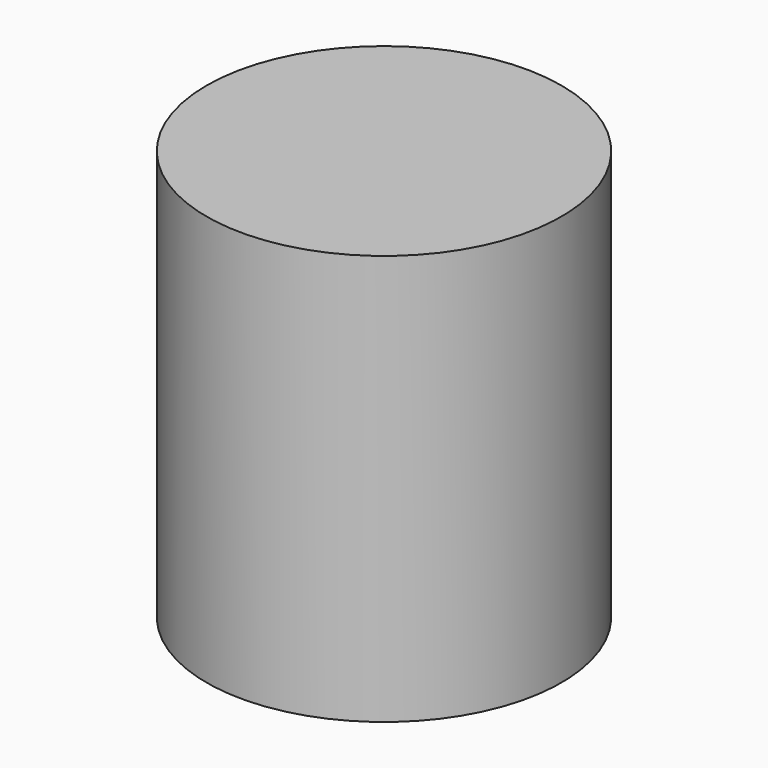
from build123d import *

# Parameters (mm, degrees)
F1_DEPTH = 25.4


# Not quite as in the source:
# - a feature names something its author has since deleted; it is built from what else it names


with BuildPart() as f1:
    # F0 (on Top) → F1 (new body)
    with BuildSketch(Plane.XY):
        with BuildLine():
            Line((0, 0), (10.9855, 0))
            ThreePointArc((10.9855, 0), (0, 10.9855), (-10.9855, 0))
            Line((-10.9855, 0), (0, 0))
        make_face()
        with BuildLine():
            ThreePointArc((-10.9855, 0), (0, -10.9855), (10.9855, 0))
            Line((10.9855, 0), (0, 0))
            Line((0, 0), (-10.9855, 0))
        make_face()
    extrude(amount=F1_DEPTH)


solid = f1.part
